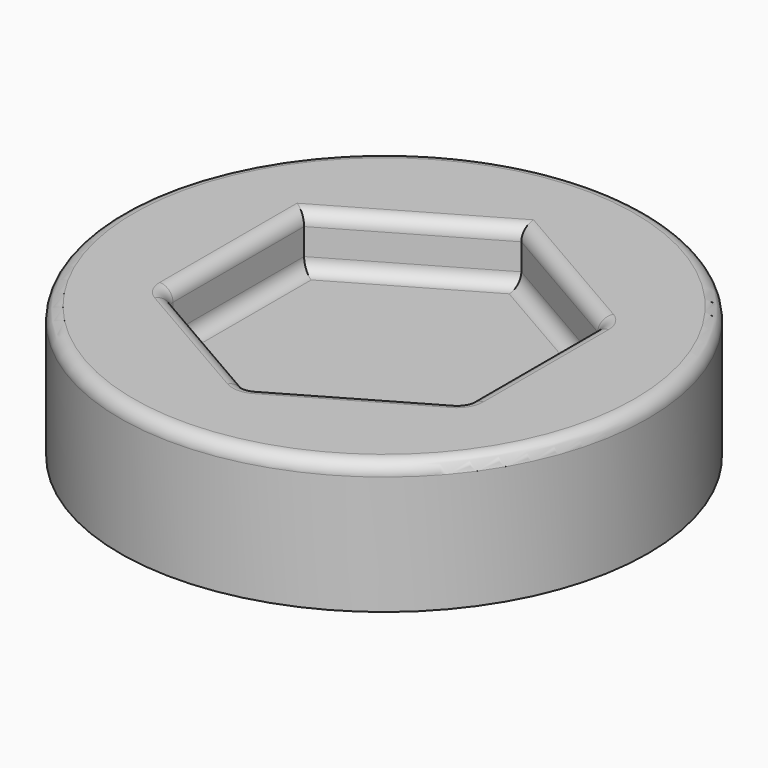
from build123d import *

# Parameters (mm, degrees)
F0_R     = 5
F1_DEPTH = 2.5
F3_DEPTH = 1
F4_R     = 0.25


with BuildPart() as f1:
    # F0 (on Top) → F1 (new body)
    with BuildSketch(Plane.XY):
        Circle(F0_R)
    extrude(amount=F1_DEPTH)

    # F2 (on face) → F3 (cut)
    with BuildSketch(Plane.XY.offset(2.5)):
        Polygon((-2.8145825623, -1.625), (0, -3.25), (2.8145825623, -1.625), (2.8145825623, 1.625), (0, 3.25), (-2.8145825623, 1.625), align=None)
    extrude(amount=-F3_DEPTH, mode=Mode.SUBTRACT)

    # F4
    f4_edges = [f1.edges().sort_by_distance(p)[0] for p in [
        (-1.407291, -2.4375, 1.5),
        (1.407291, -2.4375, 1.5),
        (2.814583, 0, 1.5),
        (1.407291, 2.4375, 1.5),
        (-1.407291, 2.4375, 1.5),
        (-2.814583, 0, 1.5),
        (2.814583, -1.625, 2),
        (2.814583, 1.625, 2),
        (2.814583, 0, 2.5),
        (-1.407291, 2.4375, 2.5),
        (-2.814583, 0, 2.5),
        (-2.814583, -1.625, 2),
        (0, -3.25, 2),
        (-1.407291, -2.4375, 2.5),
        (1.407291, -2.4375, 2.5),
        (-5, 0, 2.5),
        (1.407291, 2.4375, 2.5),
    ]]
    fillet(f4_edges, radius=F4_R)


solid = f1.part
